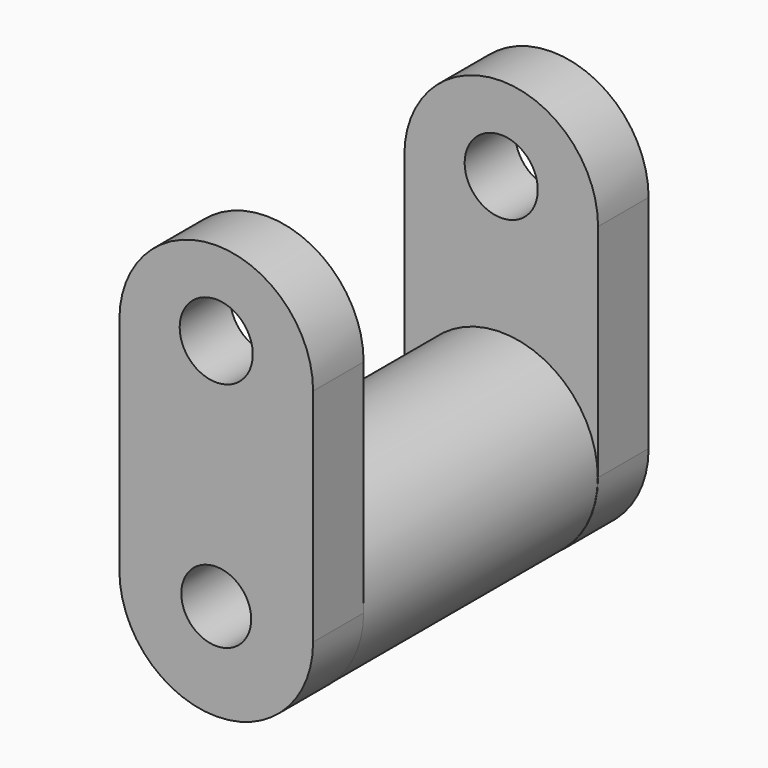
from build123d import *

# Parameters (mm, degrees)
F1_DEPTH  = 38.1
F2_W      = 53.239736706
F2_H      = 40.1604212821
F3_DEPTH  = 50.8
F4_R      = 17.5474664262
F5_DEPTH  = 38.1
F9_D      = 12.7
F10_R     = 6.6436508829
F11_DEPTH = 127


# Not quite as in the source:
# - a feature of the source that left no trace in its solid (it failed there, or was rolled back) is left out


with BuildPart() as f1:
    # F0 (on Front) → F1 (new body, symmetric)
    with BuildSketch(Plane.XZ):
        with BuildLine():
            ThreePointArc((-17.5968260456, 40.1604212821), (0, 22.5635952364), (17.5968260456, 40.1604212821))
            ThreePointArc((17.5968260456, 40.1604212821), (0, 57.7572473277), (-17.5968260456, 40.1604212821))
        make_face()
        with BuildLine():
            ThreePointArc((-17.5968260456, 0), (0, -17.5968260456), (17.5968260456, 0))
            ThreePointArc((17.5968260456, 0), (0, 17.5968260456), (-17.5968260456, 0))
        make_face()
        with BuildLine():
            ThreePointArc((-17.5968260456, 0), (0, 17.5968260456), (17.5968260456, 0))
            Line((17.5968260456, 0), (17.5968260456, 40.1604212821))
            ThreePointArc((17.5968260456, 40.1604212821), (0, 22.5635952364), (-17.5968260456, 40.1604212821))
            Line((-17.5968260456, 40.1604212821), (-17.5968260456, 0))
        make_face()
    extrude(amount=F1_DEPTH, both=True)

    # F2 (on face) → F3 (cut)
    with BuildSketch(Plane.YZ.offset(17.5968260456)):
        Polygon((0, 66.9256597757), (-26.619868353, 66.9256597757), (-26.619868353, 40.1604212821), (26.619868353, 40.1604212821), (26.619868353, 66.9256597757), align=None)
        with Locations((0, 20.080210641)):
            Rectangle(F2_W, F2_H)
        Polygon((26.619868353, 0), (-26.619868353, 0), (-26.619868353, -26.9206576049), (0, -26.9206576049), (26.619868353, -26.9206576049), align=None)
    extrude(amount=-F3_DEPTH, mode=Mode.SUBTRACT)

    # F4 (on Front) → F5 (join, symmetric)
    with BuildSketch(Plane.XZ):
        Circle(F4_R)
    extrude(amount=F5_DEPTH, both=True)

    # F9 (through all)
    with Locations(Plane.XZ.offset(38.1)):
        with Locations((0, 0)):
            Hole(F9_D / 2)

    # F10 (on face) → F11 (cut)
    with BuildSketch(Plane(origin=(0, 38.1, 0), x_dir=(-1, 0, 0), z_dir=(0, 1, 0))):
        with Locations((0, 42.4637757242)):
            Circle(F10_R)
    extrude(amount=-F11_DEPTH, mode=Mode.SUBTRACT)


solid = f1.part
